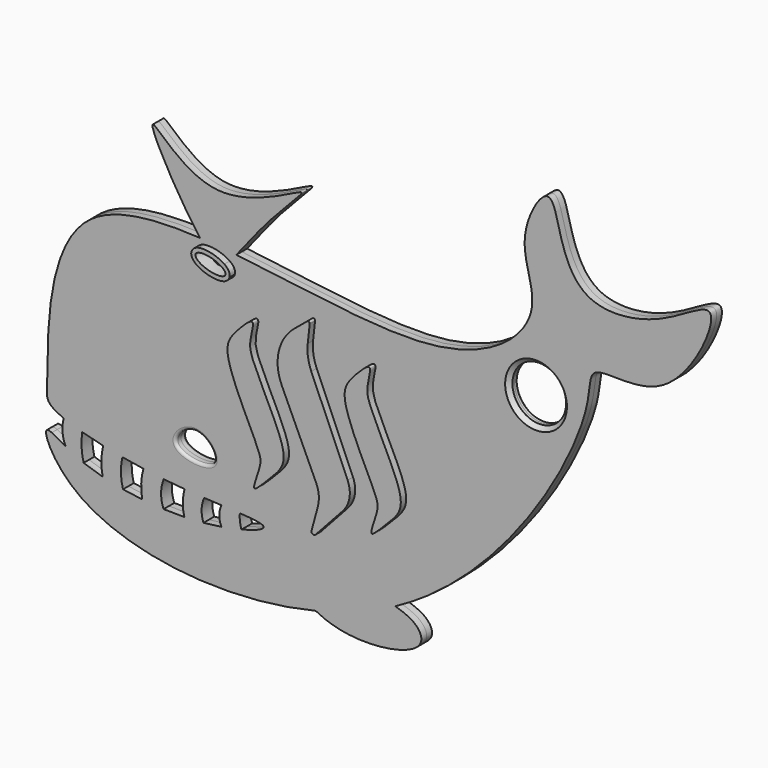
from build123d import *

# Parameters (mm, degrees)
F0_R     = 2
F1_DEPTH = 0.5
F2_DEPTH = 1
F3_R     = 0.2
F4_SIZE  = 0.3


# Not quite as in the source:
# - the dataset's text gives a spline's control points without its knots; the knots are read off the source's solid


with BuildPart() as f1:
    # F0 (on Front) → F1 (new body, symmetric)
    with BuildSketch(Plane.XZ):
        with BuildLine():
            add(Edge.make_bspline(
                [(-22.5192310189, -13.7938854355), (-22.2693112282, -13.9112969169), (-21.9162379891, -14.1367515845), (-21.4790391681, -14.3801367039)],
                knots=[0.7609203484, 0.7609203484, 0.7609203484, 0.7609203484, 0.7733390271, 0.7733390271, 0.7733390271, 0.7733390271], degree=3))
            add(Edge.make_bspline(
                [(-2.8776263382, -19.0824063202), (-9.6522427724, -20.7342049383), (-20.8738732977, -19.3002052962), (-23.3643694305, -13.5635613463), (-22.7032478457, -13.707434946), (-22.5192310189, -13.7938854355)],
                knots=[0.646912268, 0.646912268, 0.646912268, 0.646912268, 0.7137261619, 0.7517764312, 0.7609203484, 0.7609203484, 0.7609203484, 0.7609203484], degree=3))
            add(Edge.make_bspline(
                [(-5.3422385827, -13.2508724928), (-5.7040290179, -14.2334591608), (-6.1924310675, -16.108005929), (-4.2912250392, -18.3443745346), (-2.8776263382, -19.0824063202)],
                knots=[0, 0, 0, 0, 0.1499203159, 0.3050198827, 0.3050198827, 0.3050198827, 0.3050198827], degree=3))
            ThreePointArc((-5.3422385827, -13.2508724928), (-2.9770543333, -14.0544663629), (-0.5260679996, -13.5722572448))
            add(Edge.make_bspline(
                [(3.0558740018, -16.8516781591), (2.2119242086, -16.5948849601), (0.0725830758, -16.134235653), (-0.2207804001, -14.5793401417), (-0.5260679996, -13.5722572448)],
                knots=[0.7444206533, 0.7444206533, 0.7444206533, 0.7444206533, 0.8557933084, 1, 1, 1, 1], degree=3))
            add(Edge.make_bspline(
                [(-8.7802114723, 2.3285679126), (-3.789601587, 1.7997588438), (7.810309453, -0.4311737517), (14.7390968635, 5.5042876029), (11.7273009384, 10.0351269138), (14.6280033929, 15.1276172054), (15.3123166291, 10.9880777489), (17.0146945772, 7.1545001428), (22.8809603021, 7.8187435519), (28.168420429, 12.0808579173), (23.7919706234, 2.1957777822), (17.1765007208, 4.2255719819), (18.1147597255, -0.2021824516), (11.1295316199, -12.4765903359), (3.1465981315, -16.8033092101), (3.0558740018, -16.8516781591)],
                knots=[0.1056118616, 0.1056118616, 0.1056118616, 0.1056118616, 0.1536363254, 0.207703381, 0.2463087268, 0.2807742342, 0.3095878457, 0.3452519007, 0.3881086266, 0.4229361252, 0.4699208733, 0.510816889, 0.5400946169, 0.6257230641, 0.6267036504, 0.6267036504, 0.6267036504, 0.6267036504], degree=3))
            add(Edge.make_bspline(
                [(-8.7802114736, 2.3285679179), (-8.9583943308, 2.1124641386), (-9.1239169261, 1.9202832305), (-9.2751582534, 1.7598914276)],
                knots=[0.8824518348, 0.8824518348, 0.8824518348, 0.8824518348, 0.9107712064, 0.9107712064, 0.9107712064, 0.9107712064], degree=3))
            add(Edge.make_bspline(
                [(-8.8926199724, 1.0146188218), (-8.8818866058, 1.0539744956), (-8.8706128445, 1.135465745), (-8.8871946336, 1.2911661587), (-8.9604599528, 1.4545672984), (-9.087645091, 1.6096112463), (-9.2005133908, 1.7057860856), (-9.2667276435, 1.753885224), (-9.2751582534, 1.7598914276)],
                knots=[0, 0, 0, 0, 0.015625, 0.03125, 0.0625, 0.09375, 0.125, 0.1295018898, 0.1295018898, 0.1295018898, 0.1295018898], degree=3))
            add(Edge.make_bspline(
                [(-11.2061441254, 2.2051567524), (-11.220778168, 2.2018445264), (-11.3013166535, 2.1820331337), (-11.4406290966, 2.1309771257), (-11.5867074934, 2.0273970049), (-11.6800412506, 1.901673561), (-11.727530808, 1.7877763919), (-11.74444145, 1.6655395179), (-11.7278596609, 1.5098391042), (-11.6545943416, 1.3464379645), (-11.5274092035, 1.1913940166), (-11.3694822682, 1.0568248094), (-11.1841045791, 0.9370131615), (-10.9058459402, 0.7953644517), (-10.5110042017, 0.6544201655), (-10.0992765314, 0.5753909568), (-9.7876320523, 0.5561569836), (-9.5670945908, 0.5652644896), (-9.362714709, 0.6010227377), (-9.1744251978, 0.6700281372), (-9.028346801, 0.773608258), (-8.9350130438, 0.8993317019), (-8.9033533389, 0.9752631479), (-8.8926199724, 1.0146188218)],
                knots=[0.3993858518, 0.3993858518, 0.3993858518, 0.3993858518, 0.40625, 0.4375, 0.46875, 0.484375, 0.5, 0.515625, 0.53125, 0.5625, 0.59375, 0.625, 0.65625, 0.6875, 0.75, 0.8125, 0.84375, 0.875, 0.90625, 0.9375, 0.96875, 0.984375, 1, 1, 1, 1], degree=3))
            add(Edge.make_bspline(
                [(-11.2061441254, 2.2051567524), (-11.2957273193, 2.3149049209), (-11.3880633617, 2.432124368), (-11.4825226008, 2.5557213463)],
                knots=[0.0445007532, 0.0445007532, 0.0445007532, 0.0445007532, 0.0579426383, 0.0579426383, 0.0579426383, 0.0579426383], degree=3))
            add(Edge.make_bspline(
                [(-22.8618694512, -10.4405833941), (-22.7799376633, -7.9836653183), (-23.269740916, 2.0222593414), (-14.8719692595, 2.7480854153), (-11.4825226001, 2.5557213478)],
                knots=[0, 0, 0, 0, 0.0625075852, 0.096752481, 0.096752481, 0.096752481, 0.096752481], degree=3))
            add(Edge.make_bspline(
                [(-22.5192310189, -12.0846592475), (-22.9793732493, -11.7198601196), (-22.8925998629, -11.3621073311), (-22.8618694512, -10.4405833941)],
                knots=[0.9765550848, 0.9765550848, 0.9765550848, 0.9765550848, 1, 1, 1, 1], degree=3))
            add(Edge.make_bspline(
                [(-21.6285917977, -12.5611174614), (-22.0154697473, -12.4033401247), (-22.3190864776, -12.2433331297), (-22.5192310189, -12.0846592475)],
                knots=[0.9663574296, 0.9663574296, 0.9663574296, 0.9663574296, 0.9765550848, 0.9765550848, 0.9765550848, 0.9765550848], degree=3))
            add(Edge.make_bspline(
                [(-20.2537305215, -13.0198812448), (-20.7805977101, -12.871454419), (-21.2454295383, -12.7173794579), (-21.6285917977, -12.5611174614)],
                knots=[0.9562577157, 0.9562577157, 0.9562577157, 0.9562577157, 0.9663574296, 0.9663574296, 0.9663574296, 0.9663574296], degree=3))
            add(Edge.make_bspline(
                [(-18.6952734305, -13.4042731031), (-19.2554434468, -13.2823952036), (-19.7796958566, -13.1534243125), (-20.2537305215, -13.0198812448)],
                knots=[0.9471707682, 0.9471707682, 0.9471707682, 0.9471707682, 0.9562577157, 0.9562577157, 0.9562577157, 0.9562577157], degree=3))
            add(Edge.make_bspline(
                [(-17.2619816869, -13.6867383116), (-17.7584387677, -13.5982030729), (-18.2387823063, -13.5035932697), (-18.6952734305, -13.4042731031)],
                knots=[0.9397656755, 0.9397656755, 0.9397656755, 0.9397656755, 0.9471707682, 0.9471707682, 0.9471707682, 0.9471707682], degree=3))
            add(Edge.make_bspline(
                [(-15.7004295414, -13.937293297), (-16.2322397673, -13.861063123), (-16.7554962758, -13.7770619438), (-17.2619816869, -13.6867383116)],
                knots=[0.9322110015, 0.9322110015, 0.9322110015, 0.9322110015, 0.9397656755, 0.9397656755, 0.9397656755, 0.9397656755], degree=3))
            add(Edge.make_bspline(
                [(-14.1835960649, -14.1306026721), (-14.6922163648, -14.0738483232), (-15.200108332, -14.009009806), (-15.7004295414, -13.937293297)],
                knots=[0.9251036473, 0.9251036473, 0.9251036473, 0.9251036473, 0.9322110015, 0.9322110015, 0.9322110015, 0.9322110015], degree=3))
            add(Edge.make_bspline(
                [(-12.635330315, -14.2778200216), (-12.8398046392, -14.2616452056), (-13.3545059481, -14.2180365227), (-13.8727863625, -14.1652843438), (-14.1835960649, -14.1306026721)],
                knots=[0.9178676366, 0.9178676366, 0.9178676366, 0.9178676366, 0.9207604572, 0.9251036473, 0.9251036473, 0.9251036473, 0.9251036473], degree=3))
            add(Edge.make_bspline(
                [(-11.1786203575, -14.3762945075), (-11.6496662931, -14.3489658391), (-12.1386826121, -14.3171070337), (-12.635330315, -14.2778200216)],
                knots=[0.9108412644, 0.9108412644, 0.9108412644, 0.9108412644, 0.9178676366, 0.9178676366, 0.9178676366, 0.9178676366], degree=3))
            add(Edge.make_bspline(
                [(-9.8935888984, -14.4444040798), (-10.2998019757, -14.424133033), (-10.7311011027, -14.4022582286), (-11.1786203575, -14.3762945075)],
                knots=[0.9041658287, 0.9041658287, 0.9041658287, 0.9041658287, 0.9108412644, 0.9108412644, 0.9108412644, 0.9108412644], degree=3))
            add(Edge.make_bspline(
                [(-8.5257092058, -14.5165079527), (-8.9327790479, -14.4918191007), (-9.3942290645, -14.4693233824), (-9.8935888984, -14.4444040798)],
                knots=[0.8959596811, 0.8959596811, 0.8959596811, 0.8959596811, 0.9041658287, 0.9041658287, 0.9041658287, 0.9041658287], degree=3))
            add(Edge.make_bspline(
                [(-8.4071998008, -15.5573212753), (-7.3900285165, -15.3038727883), (-6.0579544978, -14.7422559813), (-7.4612236956, -14.5810691716), (-8.5257092058, -14.5165079527)],
                knots=[0.8524832233, 0.8524832233, 0.8524832233, 0.8524832233, 0.874500648, 0.8959596811, 0.8959596811, 0.8959596811, 0.8959596811], degree=3))
            add(Edge.make_bspline(
                [(-9.8966210033, -15.8590198352), (-9.3551456033, -15.7715876745), (-8.8488764122, -15.6673738011), (-8.4071998008, -15.5573212753)],
                knots=[0.8429228064, 0.8429228064, 0.8429228064, 0.8429228064, 0.8524832233, 0.8524832233, 0.8524832233, 0.8524832233], degree=3))
            add(Edge.make_bspline(
                [(-11.2288753209, -16.0291895656), (-11.1941259306, -16.0259352669), (-10.7383261652, -15.9820230395), (-10.2911061499, -15.922717445), (-9.8966210033, -15.8590198352)],
                knots=[0.835383703, 0.835383703, 0.835383703, 0.835383703, 0.8359576839, 0.8429228064, 0.8429228064, 0.8429228064, 0.8429228064], degree=3))
            add(Edge.make_bspline(
                [(-12.6555407934, -16.1131222257), (-12.1748071406, -16.100795439), (-11.6975122326, -16.0730776597), (-11.2288753209, -16.0291895656)],
                knots=[0.8276428871, 0.8276428871, 0.8276428871, 0.8276428871, 0.835383703, 0.835383703, 0.835383703, 0.835383703], degree=3))
            add(Edge.make_bspline(
                [(-14.2008752796, -16.1009146707), (-13.6860790623, -16.1218988669), (-13.1688496464, -16.126284293), (-12.6555407934, -16.1131222257)],
                knots=[0.8193775424, 0.8193775424, 0.8193775424, 0.8193775424, 0.8276428871, 0.8276428871, 0.8276428871, 0.8276428871], degree=3))
            add(Edge.make_bspline(
                [(-15.7850211201, -15.9834062361), (-15.2642823801, -16.0396676506), (-14.733883029, -16.0791881335), (-14.2008752796, -16.1009146707)],
                knots=[0.8108198013, 0.8108198013, 0.8108198013, 0.8108198013, 0.8193775424, 0.8193775424, 0.8193775424, 0.8193775424], degree=3))
            add(Edge.make_bspline(
                [(-17.2175950237, -15.7820234188), (-16.7524202992, -15.8632720066), (-16.2729617142, -15.9306883837), (-15.7850211201, -15.9834062361)],
                knots=[0.8028010599, 0.8028010599, 0.8028010599, 0.8028010599, 0.8108198013, 0.8108198013, 0.8108198013, 0.8108198013], degree=3))
            add(Edge.make_bspline(
                [(-18.7347995075, -15.4539759448), (-18.2530085667, -15.5802304647), (-17.7444637519, -15.689999201), (-17.2175950237, -15.7820234188)],
                knots=[0.7937188293, 0.7937188293, 0.7937188293, 0.7937188293, 0.8028010599, 0.8028010599, 0.8028010599, 0.8028010599], degree=3))
            add(Edge.make_bspline(
                [(-20.1510576998, -15.0044054939), (-19.7147861735, -15.1713866009), (-19.2394704749, -15.3217256566), (-18.7347995075, -15.4539759448)],
                knots=[0.7842052879, 0.7842052879, 0.7842052879, 0.7842052879, 0.7937188293, 0.7937188293, 0.7937188293, 0.7937188293], degree=3))
            add(Edge.make_bspline(
                [(-21.4790391681, -14.3801367039), (-21.2603129222, -14.5018998718), (-20.8409408643, -14.7227092866), (-20.3644493632, -14.9227307248), (-20.1510576998, -15.0044054939)],
                knots=[0.7733390271, 0.7733390271, 0.7733390271, 0.7733390271, 0.7795519693, 0.7842052879, 0.7842052879, 0.7842052879, 0.7842052879], degree=3))
        make_face()
        with BuildLine():
            add(Edge.make_bspline(
                [(-13.2434293628, -11.5714259446), (-13.5252085637, -11.0194385936), (-11.7070129072, -9.2709826341), (-9.1983943803, -12.6375408621), (-12.9097713248, -12.2250406043), (-13.2434293628, -11.5714259446)],
                knots=[0, 0, 0, 0, 0.3110308456, 0.6317047484, 1, 1, 1, 1], degree=3))
        make_face(mode=Mode.SUBTRACT)
        with BuildLine():
            add(Edge.make_bspline(
                [(-7.2008277078, -1.3674281827), (-7.3670301146, -1.2695996245), (-8.627037368, -2.5424159378), (-9.604639754, -4.0531033278), (-6.6463232235, -9.5044730052), (-6.4877686794, -10.5141118358), (-7.4354522299, -12.7956934911), (-6.0152288528, -11.2873535902), (-4.7065014678, -10.09309799), (-4.9524675477, -8.1113782169), (-7.3510013808, -3.7881177406), (-7.4070508281, -2.652112134), (-7.0626654573, -1.4487519975), (-7.2008277078, -1.3674281827)],
                knots=[0, 0, 0, 0, 0.0802945363, 0.1681190554, 0.3215380874, 0.3955240052, 0.4738924268, 0.5433635783, 0.6300738878, 0.717746988, 0.8588403284, 0.9332520265, 1, 1, 1, 1], degree=3))
        make_face(mode=Mode.SUBTRACT)
        with BuildLine():
            Line((-4.0928410954, -0.7955430284), (-3.1121504583, 0.017312022))
            ThreePointArc((-3.1121504583, 0.017312022), (-2.9828262004, 0.0302091465), (-2.922257293, -0.0847800137))
            Line((-2.922257293, -0.0847800137), (-3.0673342694, -1.4242685717))
            ThreePointArc((-3.0673342694, -1.4242685717), (-3.0485301344, -2.3116617963), (-2.8038055931, -3.1648500694))
            Line((-2.8038055931, -3.1648500694), (-0.0995264069, -9.4140178702))
            ThreePointArc((-0.0995264069, -9.4140178702), (0.036385917, -10.5316535152), (-0.4571588168, -11.54357999))
            Line((-0.4571588168, -11.54357999), (-2.4862750029, -13.7605778944))
            ThreePointArc((-2.4862750029, -13.7605778944), (-2.700543815, -13.7957448089), (-2.7850176732, -13.5957148037))
            Line((-2.7850176732, -13.5957148037), (-2.321039241, -11.9018280073))
            ThreePointArc((-2.321039241, -11.9018280073), (-2.2469315732, -11.1030327178), (-2.4509835487, -10.3271921078))
            Line((-2.4509835487, -10.3271921078), (-5.0014014622, -4.7957878345))
            ThreePointArc((-5.0014014622, -4.7957878345), (-5.2270398503, -2.6412381159), (-4.0928410954, -0.7955430284))
        make_face(mode=Mode.SUBTRACT)
        with BuildLine():
            add(Edge.make_bspline(
                [(1.5199846821, -1.4996984974), (1.3537822753, -1.4018699392), (0.0937750219, -2.6746862525), (-0.8838273641, -4.1853736425), (2.0744891664, -9.6367433199), (2.2330437105, -10.6463821505), (1.28536016, -12.9279638058), (2.7055835371, -11.4196239049), (4.0143109221, -10.2253683047), (3.7683448421, -8.2436485315), (1.3698110091, -3.9203880553), (1.3137615618, -2.7843824487), (1.6581469326, -1.5810223122), (1.5199846821, -1.4996984974)],
                knots=[0, 0, 0, 0, 0.0802945363, 0.1681190554, 0.3215380874, 0.3955240052, 0.4738924268, 0.5433635783, 0.6300738878, 0.717746988, 0.8588403284, 0.9332520265, 1, 1, 1, 1], degree=3))
        make_face(mode=Mode.SUBTRACT)
        with Locations((13.5268429294, 0.3782608837)):
            Circle(F0_R, mode=Mode.SUBTRACT)
        with BuildLine():
            ThreePointArc((-21.6285917977, -12.5611174614), (-21.724608188, -13.4846689891), (-21.4790391681, -14.3801367039))
            add(Edge.make_bspline(
                [(-21.4790391681, -14.3801367039), (-21.2603129222, -14.5018998718), (-20.8409408643, -14.7227092866), (-20.3644493632, -14.9227307248), (-20.1510576998, -15.0044054939)],
                knots=[0.7733390271, 0.7733390271, 0.7733390271, 0.7733390271, 0.7795519693, 0.7842052879, 0.7842052879, 0.7842052879, 0.7842052879], degree=3))
            ThreePointArc((-20.1510576998, -15.0044054939), (-20.3013614481, -14.0172636171), (-20.2537305215, -13.0198812448))
            add(Edge.make_bspline(
                [(-20.2537305215, -13.0198812448), (-20.7805977101, -12.871454419), (-21.2454295383, -12.7173794579), (-21.6285917977, -12.5611174614)],
                knots=[0.9562577157, 0.9562577157, 0.9562577157, 0.9562577157, 0.9663574296, 0.9663574296, 0.9663574296, 0.9663574296], degree=3))
        make_face()
        with BuildLine():
            add(Edge.make_bspline(
                [(-5.3422385827, -13.2508724928), (-5.7040290179, -14.2334591608), (-6.1924310675, -16.108005929), (-4.2912250392, -18.3443745346), (-2.8776263382, -19.0824063202)],
                knots=[0, 0, 0, 0, 0.1499203159, 0.3050198827, 0.3050198827, 0.3050198827, 0.3050198827], degree=3))
            add(Edge.make_bspline(
                [(3.0558740018, -16.8516781591), (1.186166826, -17.848499747), (-0.8285670018, -18.5828011524), (-2.8776263382, -19.0824063202)],
                knots=[0.6267036504, 0.6267036504, 0.6267036504, 0.6267036504, 0.646912268, 0.646912268, 0.646912268, 0.646912268], degree=3))
            add(Edge.make_bspline(
                [(3.0558740018, -16.8516781591), (2.2119242086, -16.5948849601), (0.0725830758, -16.134235653), (-0.2207804001, -14.5793401417), (-0.5260679996, -13.5722572448)],
                knots=[0.7444206533, 0.7444206533, 0.7444206533, 0.7444206533, 0.8557933084, 1, 1, 1, 1], degree=3))
            ThreePointArc((-0.5260679996, -13.5722572448), (-2.9770543333, -14.0544663629), (-5.3422385827, -13.2508724928))
        make_face()
        with BuildLine():
            add(Edge.make_bspline(
                [(3.0558740018, -16.8516781591), (1.186166826, -17.848499747), (-0.8285670018, -18.5828011524), (-2.8776263382, -19.0824063202)],
                knots=[0.6267036504, 0.6267036504, 0.6267036504, 0.6267036504, 0.646912268, 0.646912268, 0.646912268, 0.646912268], degree=3))
            add(Edge.make_bspline(
                [(-2.8776263382, -19.0824063202), (-2.4175454507, -19.3226119165), (0.2973345884, -20.3815909392), (5.772456854, -19.4866806857), (4.7234035585, -17.4273704856), (3.5131315322, -16.9908103976), (3.0558740018, -16.8516781591)],
                knots=[0.3050198827, 0.3050198827, 0.3050198827, 0.3050198827, 0.3554998005, 0.5751078548, 0.6840782187, 0.7444206533, 0.7444206533, 0.7444206533, 0.7444206533], degree=3))
        make_face()
        with BuildLine():
            ThreePointArc((-18.6952734305, -13.4042731031), (-18.8294837702, -14.4269175441), (-18.7347995075, -15.4539759448))
            add(Edge.make_bspline(
                [(-18.7347995075, -15.4539759448), (-18.2530085667, -15.5802304647), (-17.7444637519, -15.689999201), (-17.2175950237, -15.7820234188)],
                knots=[0.7937188293, 0.7937188293, 0.7937188293, 0.7937188293, 0.8028010599, 0.8028010599, 0.8028010599, 0.8028010599], degree=3))
            ThreePointArc((-17.2175950237, -15.7820234188), (-17.373442176, -14.7372121969), (-17.2619816869, -13.6867383116))
            add(Edge.make_bspline(
                [(-17.2619816869, -13.6867383116), (-17.7584387677, -13.5982030729), (-18.2387823063, -13.5035932697), (-18.6952734305, -13.4042731031)],
                knots=[0.9397656755, 0.9397656755, 0.9397656755, 0.9397656755, 0.9471707682, 0.9471707682, 0.9471707682, 0.9471707682], degree=3))
        make_face()
        with BuildLine():
            add(Edge.make_bspline(
                [(-8.7802114736, 2.3285679179), (-8.9583943308, 2.1124641386), (-9.1239169261, 1.9202832305), (-9.2751582534, 1.7598914276)],
                knots=[0.8824518348, 0.8824518348, 0.8824518348, 0.8824518348, 0.9107712064, 0.9107712064, 0.9107712064, 0.9107712064], degree=3))
            add(Edge.make_bspline(
                [(-11.4825226001, 2.5557213478), (-10.6056503746, 2.5059554937), (-9.7008612592, 2.4261207103), (-8.7802114723, 2.3285679126)],
                knots=[0.096752481, 0.096752481, 0.096752481, 0.096752481, 0.1056118616, 0.1056118616, 0.1056118616, 0.1056118616], degree=3))
            add(Edge.make_bspline(
                [(-11.2061441254, 2.2051567524), (-11.2957273193, 2.3149049209), (-11.3880633617, 2.432124368), (-11.4825226008, 2.5557213463)],
                knots=[0.0445007532, 0.0445007532, 0.0445007532, 0.0445007532, 0.0579426383, 0.0579426383, 0.0579426383, 0.0579426383], degree=3))
            add(Edge.make_bspline(
                [(-9.2751582534, 1.7598914276), (-9.3252489697, 1.7955774628), (-9.4409712331, 1.8690935964), (-9.7092083542, 2.0056408111), (-10.1040500928, 2.1465850974), (-10.5157777631, 2.2256143061), (-10.8274222422, 2.2448482793), (-11.0318124843, 2.2364076028), (-11.1541546307, 2.2169239015), (-11.2061441254, 2.2051567524)],
                knots=[0.1295018898, 0.1295018898, 0.1295018898, 0.1295018898, 0.15625, 0.1875, 0.25, 0.3125, 0.34375, 0.375, 0.3993858518, 0.3993858518, 0.3993858518, 0.3993858518], degree=3))
        make_face()
        with BuildLine():
            add(Edge.make_bspline(
                [(-11.4825226001, 2.5557213478), (-10.6056503746, 2.5059554937), (-9.7008612592, 2.4261207103), (-8.7802114723, 2.3285679126)],
                knots=[0.096752481, 0.096752481, 0.096752481, 0.096752481, 0.1056118616, 0.1056118616, 0.1056118616, 0.1056118616], degree=3))
            add(Edge.make_bspline(
                [(-11.4825226008, 2.5557213463), (-12.3641492131, 3.7093023651), (-14.3355139975, 6.8683100237), (-15.8021837386, 10.334426695), (-10.6498763228, 3.801175625), (-1.8895443974, 9.6004007768), (-6.1317297679, 5.8283793726), (-8.0807106624, 3.1769366742), (-8.7802114736, 2.3285679179)],
                knots=[0.0579426383, 0.0579426383, 0.0579426383, 0.0579426383, 0.1834012356, 0.2898275669, 0.4560378407, 0.6402498697, 0.7712771473, 0.8824518348, 0.8824518348, 0.8824518348, 0.8824518348], degree=3))
        make_face()
        with BuildLine():
            ThreePointArc((-15.7004295414, -13.937293297), (-15.861984421, -14.9554192886), (-15.7850211201, -15.9834062361))
            add(Edge.make_bspline(
                [(-15.7850211201, -15.9834062361), (-15.2642823801, -16.0396676506), (-14.733883029, -16.0791881335), (-14.2008752796, -16.1009146707)],
                knots=[0.8108198013, 0.8108198013, 0.8108198013, 0.8108198013, 0.8193775424, 0.8193775424, 0.8193775424, 0.8193775424], degree=3))
            ThreePointArc((-14.2008752796, -16.1009146707), (-14.3852613408, -15.1140658776), (-14.1835960649, -14.1306026721))
            add(Edge.make_bspline(
                [(-14.1835960649, -14.1306026721), (-14.6922163648, -14.0738483232), (-15.200108332, -14.009009806), (-15.7004295414, -13.937293297)],
                knots=[0.9251036473, 0.9251036473, 0.9251036473, 0.9251036473, 0.9322110015, 0.9322110015, 0.9322110015, 0.9322110015], degree=3))
        make_face()
        with BuildLine():
            ThreePointArc((-12.635330315, -14.2778200216), (-12.7673590022, -15.194128494), (-12.6555407934, -16.1131222257))
            add(Edge.make_bspline(
                [(-12.6555407934, -16.1131222257), (-12.1748071406, -16.100795439), (-11.6975122326, -16.0730776597), (-11.2288753209, -16.0291895656)],
                knots=[0.8276428871, 0.8276428871, 0.8276428871, 0.8276428871, 0.835383703, 0.835383703, 0.835383703, 0.835383703], degree=3))
            ThreePointArc((-11.2288753209, -16.0291895656), (-11.3674846768, -15.1977637479), (-11.1786203575, -14.3762945075))
            add(Edge.make_bspline(
                [(-11.1786203575, -14.3762945075), (-11.6496662931, -14.3489658391), (-12.1386826121, -14.3171070337), (-12.635330315, -14.2778200216)],
                knots=[0.9108412644, 0.9108412644, 0.9108412644, 0.9108412644, 0.9178676366, 0.9178676366, 0.9178676366, 0.9178676366], degree=3))
        make_face()
        with BuildLine():
            ThreePointArc((-9.8935888984, -14.4444040798), (-10.0470740326, -15.1513862251), (-9.8966210033, -15.8590198352))
            add(Edge.make_bspline(
                [(-9.8966210033, -15.8590198352), (-9.3551456033, -15.7715876745), (-8.8488764122, -15.6673738011), (-8.4071998008, -15.5573212753)],
                knots=[0.8429228064, 0.8429228064, 0.8429228064, 0.8429228064, 0.8524832233, 0.8524832233, 0.8524832233, 0.8524832233], degree=3))
            ThreePointArc((-8.4071998008, -15.5573212753), (-8.5167447557, -15.0426407781), (-8.5257092058, -14.5165079527))
            add(Edge.make_bspline(
                [(-8.5257092058, -14.5165079527), (-8.9327790479, -14.4918191007), (-9.3942290645, -14.4693233824), (-9.8935888984, -14.4444040798)],
                knots=[0.8959596811, 0.8959596811, 0.8959596811, 0.8959596811, 0.9041658287, 0.9041658287, 0.9041658287, 0.9041658287], degree=3))
        make_face()
    extrude(amount=F1_DEPTH, both=True)



with BuildPart() as f1b:
    # F0 (on Front) → F1, piece 2 (new body, symmetric)
    with BuildSketch(Plane.XZ):
        with BuildLine():
            add(Edge.make_bspline(
                [(-9.4985694796, 1.537229838), (-9.5549075693, 1.4853133173), (-9.8964531421, 1.194489379), (-10.1285492057, 1.1748095892), (-10.4297818616, 1.4005026314)],
                knots=[0.9254478267, 0.9254478267, 0.9254478267, 0.9254478267, 0.93717886, 1, 1, 1, 1], degree=3))
            add(Edge.make_bspline(
                [(-9.4985694796, 1.537229838), (-10.1787298227, 1.985622169), (-10.9705402704, 1.9267938894)],
                knots=[0.8714905565, 0.8714905565, 0.8714905565, 2.3087570714, 2.3087570714, 2.3087570714], degree=2, weights=[1, 0.7527062358, 1]))
            add(Edge.make_bspline(
                [(-10.4297818616, 1.4005026314), (-10.584933046, 1.5167468106), (-10.7681132024, 1.697262241), (-10.9705402704, 1.9267938894)],
                knots=[0, 0, 0, 0, 0.0323563003, 0.0323563003, 0.0323563003, 0.0323563003], degree=3))
        make_face()
    extrude(amount=F1_DEPTH, both=True)


with BuildPart() as f2:
    # F0 (on Front) → F2 (new body, symmetric)
    with BuildSketch(Plane.XZ):
        with BuildLine():
            add(Edge.make_bspline(
                [(-7.2008277078, -1.3674281827), (-7.3670301146, -1.2695996245), (-8.627037368, -2.5424159378), (-9.604639754, -4.0531033278), (-6.6463232235, -9.5044730052), (-6.4877686794, -10.5141118358), (-7.4354522299, -12.7956934911), (-6.0152288528, -11.2873535902), (-4.7065014678, -10.09309799), (-4.9524675477, -8.1113782169), (-7.3510013808, -3.7881177406), (-7.4070508281, -2.652112134), (-7.0626654573, -1.4487519975), (-7.2008277078, -1.3674281827)],
                knots=[0, 0, 0, 0, 0.0802945363, 0.1681190554, 0.3215380874, 0.3955240052, 0.4738924268, 0.5433635783, 0.6300738878, 0.717746988, 0.8588403284, 0.9332520265, 1, 1, 1, 1], degree=3))
        make_face()
    extrude(amount=F2_DEPTH, both=True)


with BuildPart() as f2b:
    # F0 (on Front) → F2, piece 2 (new body, symmetric)
    with BuildSketch(Plane.XZ):
        with BuildLine():
            ThreePointArc((-2.922257293, -0.0847800137), (-2.9828262004, 0.0302091465), (-3.1121504583, 0.017312022))
            Line((-3.1121504583, 0.017312022), (-4.0928410954, -0.7955430284))
            ThreePointArc((-4.0928410954, -0.7955430284), (-5.2270398503, -2.6412381159), (-5.0014014622, -4.7957878345))
            Line((-5.0014014622, -4.7957878345), (-2.4509835487, -10.3271921078))
            ThreePointArc((-2.4509835487, -10.3271921078), (-2.2469315732, -11.1030327178), (-2.321039241, -11.9018280073))
            Line((-2.321039241, -11.9018280073), (-2.7850176732, -13.5957148037))
            ThreePointArc((-2.7850176732, -13.5957148037), (-2.700543815, -13.7957448089), (-2.4862750029, -13.7605778944))
            Line((-2.4862750029, -13.7605778944), (-0.4571588168, -11.54357999))
            ThreePointArc((-0.4571588168, -11.54357999), (0.036385917, -10.5316535152), (-0.0995264069, -9.4140178702))
            Line((-0.0995264069, -9.4140178702), (-2.8038055931, -3.1648500694))
            ThreePointArc((-2.8038055931, -3.1648500694), (-3.0485301344, -2.3116617963), (-3.0673342694, -1.4242685717))
            Line((-3.0673342694, -1.4242685717), (-2.922257293, -0.0847800137))
        make_face()
    extrude(amount=F2_DEPTH, both=True)


with BuildPart() as f2c:
    # F0 (on Front) → F2, piece 3 (new body, symmetric)
    with BuildSketch(Plane.XZ):
        with BuildLine():
            add(Edge.make_bspline(
                [(1.5199846821, -1.4996984974), (1.3537822753, -1.4018699392), (0.0937750219, -2.6746862525), (-0.8838273641, -4.1853736425), (2.0744891664, -9.6367433199), (2.2330437105, -10.6463821505), (1.28536016, -12.9279638058), (2.7055835371, -11.4196239049), (4.0143109221, -10.2253683047), (3.7683448421, -8.2436485315), (1.3698110091, -3.9203880553), (1.3137615618, -2.7843824487), (1.6581469326, -1.5810223122), (1.5199846821, -1.4996984974)],
                knots=[0, 0, 0, 0, 0.0802945363, 0.1681190554, 0.3215380874, 0.3955240052, 0.4738924268, 0.5433635783, 0.6300738878, 0.717746988, 0.8588403284, 0.9332520265, 1, 1, 1, 1], degree=3))
        make_face()
    extrude(amount=F2_DEPTH, both=True)


with BuildPart() as f1_1:
    add(f1.part)

    add(f1b.part)  # F2#4 merges F1b
    # F0 (on Front) → F2, piece 4 (join, symmetric)
    with BuildSketch(Plane.XZ):
        with BuildLine():
            add(Edge.make_bspline(
                [(-9.2751582534, 1.7598914276), (-9.3535396368, 1.676767776), (-9.4280852581, 1.6021822629), (-9.4985694796, 1.537229838)],
                knots=[0.9107712064, 0.9107712064, 0.9107712064, 0.9107712064, 0.9254478267, 0.9254478267, 0.9254478267, 0.9254478267], degree=3))
            add(Edge.make_bspline(
                [(-9.2751582534, 1.7598914276), (-9.3252489697, 1.7955774628), (-9.4409712331, 1.8690935964), (-9.7092083542, 2.0056408111), (-10.1040500928, 2.1465850974), (-10.5157777631, 2.2256143061), (-10.8274222422, 2.2448482793), (-11.0318124843, 2.2364076028), (-11.1541546307, 2.2169239015), (-11.2061441254, 2.2051567524)],
                knots=[0.1295018898, 0.1295018898, 0.1295018898, 0.1295018898, 0.15625, 0.1875, 0.25, 0.3125, 0.34375, 0.375, 0.3993858518, 0.3993858518, 0.3993858518, 0.3993858518], degree=3))
            add(Edge.make_bspline(
                [(-10.9705402704, 1.9267938894), (-11.0465182397, 2.0129451571), (-11.1252076443, 2.1060016524), (-11.2061441254, 2.2051567524)],
                knots=[0.0323563003, 0.0323563003, 0.0323563003, 0.0323563003, 0.0445007532, 0.0445007532, 0.0445007532, 0.0445007532], degree=3))
            add(Edge.make_bspline(
                [(-9.4985694796, 1.537229838), (-10.1787298227, 1.985622169), (-10.9705402704, 1.9267938894)],
                knots=[0.8714905565, 0.8714905565, 0.8714905565, 2.3087570714, 2.3087570714, 2.3087570714], degree=2, weights=[1, 0.7527062358, 1]))
        make_face()
        with BuildLine():
            add(Edge.make_bspline(
                [(-8.8926199724, 1.0146188218), (-8.8818866058, 1.0539744956), (-8.8706128445, 1.135465745), (-8.8871946336, 1.2911661587), (-8.9604599528, 1.4545672984), (-9.087645091, 1.6096112463), (-9.2005133908, 1.7057860856), (-9.2667276435, 1.753885224), (-9.2751582534, 1.7598914276)],
                knots=[0, 0, 0, 0, 0.015625, 0.03125, 0.0625, 0.09375, 0.125, 0.1295018898, 0.1295018898, 0.1295018898, 0.1295018898], degree=3))
            add(Edge.make_bspline(
                [(-9.2751582534, 1.7598914276), (-9.3535396368, 1.676767776), (-9.4280852581, 1.6021822629), (-9.4985694796, 1.537229838)],
                knots=[0.9107712064, 0.9107712064, 0.9107712064, 0.9107712064, 0.9254478267, 0.9254478267, 0.9254478267, 0.9254478267], degree=3))
            add(Edge.make_bspline(
                [(-9.1916964499, 1.0961851412), (-9.1365080389, 1.29854263), (-9.4985694796, 1.537229838)],
                knots=[0, 0, 0, 0.8714905565, 0.8714905565, 0.8714905565], degree=2, weights=[1, 0.9065557225, 1]))
            add(Edge.make_bspline(
                [(-10.9705402704, 1.9267938894), (-12.3608091951, 1.8235025912), (-10.8672702409, 1.1261133619), (-9.3737312868, 0.4287241326), (-9.1916964499, 1.0961851412)],
                knots=[2.3087570714, 2.3087570714, 2.3087570714, 4.2959711893, 4.2959711893, 6.2831853072, 6.2831853072, 6.2831853072], degree=2, weights=[1, 0.5456707027, 1, 0.5456707027, 1]))
            add(Edge.make_bspline(
                [(-10.9705402704, 1.9267938894), (-11.0465182397, 2.0129451571), (-11.1252076443, 2.1060016524), (-11.2061441254, 2.2051567524)],
                knots=[0.0323563003, 0.0323563003, 0.0323563003, 0.0323563003, 0.0445007532, 0.0445007532, 0.0445007532, 0.0445007532], degree=3))
            add(Edge.make_bspline(
                [(-11.2061441254, 2.2051567524), (-11.220778168, 2.2018445264), (-11.3013166535, 2.1820331337), (-11.4406290966, 2.1309771257), (-11.5867074934, 2.0273970049), (-11.6800412506, 1.901673561), (-11.727530808, 1.7877763919), (-11.74444145, 1.6655395179), (-11.7278596609, 1.5098391042), (-11.6545943416, 1.3464379645), (-11.5274092035, 1.1913940166), (-11.3694822682, 1.0568248094), (-11.1841045791, 0.9370131615), (-10.9058459402, 0.7953644517), (-10.5110042017, 0.6544201655), (-10.0992765314, 0.5753909568), (-9.7876320523, 0.5561569836), (-9.5670945908, 0.5652644896), (-9.362714709, 0.6010227377), (-9.1744251978, 0.6700281372), (-9.028346801, 0.773608258), (-8.9350130438, 0.8993317019), (-8.9033533389, 0.9752631479), (-8.8926199724, 1.0146188218)],
                knots=[0.3993858518, 0.3993858518, 0.3993858518, 0.3993858518, 0.40625, 0.4375, 0.46875, 0.484375, 0.5, 0.515625, 0.53125, 0.5625, 0.59375, 0.625, 0.65625, 0.6875, 0.75, 0.8125, 0.84375, 0.875, 0.90625, 0.9375, 0.96875, 0.984375, 1, 1, 1, 1], degree=3))
        make_face()
    extrude(amount=F2_DEPTH, both=True)

    # F3
    f3_edges = [f1_1.edges().sort_by_distance(p)[0] for p in [
        (-10.55194, -0.5, -11.099359),
        (-10.55194, 0.5, -11.099359),
    ]]
    fillet(f3_edges, radius=F3_R)

    # F4
    f4_edges = [f1_1.edges().sort_by_distance(p)[0] for p in [
        (11.526843, -0.5, 0.378261),
        (11.526843, 0.5, 0.378261),
    ]]
    chamfer(f4_edges, length=F4_SIZE)


solid = Compound([f2.part, f2b.part, f2c.part, f1_1.part])
